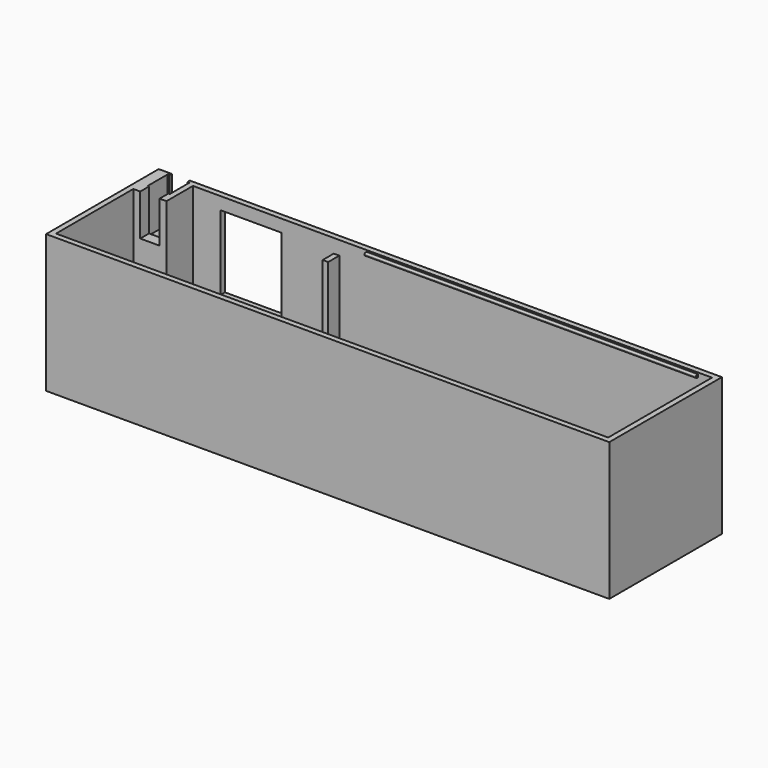
from build123d import *

# Parameters (mm, degrees)
F1_DEPTH  = 2
F0_W      = 204
F0_H      = 51
F0_W_2    = 12
F0_H_2    = 12
F2_DEPTH  = 50
F0_W_3    = 2
F0_H_3    = 37
F3_DEPTH  = 7
F0_H_4    = 5
F4_DEPTH  = 45
F6_DEPTH  = 16
F5_W      = 7
F5_H      = 4
F7_DEPTH  = 15
F8_W      = 22
F8_H      = 27
F9_DEPTH  = 5
F10_W     = 120
F10_H     = 1
F11_DEPTH = 3
F12_W     = 120
F12_H     = 1
F13_DEPTH = 3
F14_R     = 0.4


# Not quite as in the source:
# - a feature names something its author has since deleted; it is built from what else it names


with BuildPart() as f1:
    # F0 (on Top) → F1 (new body)
    with BuildSketch(Plane.XY):
        Polygon((200, 0), (65, 0), (65, -5), (65, -42), (65, -47), (200, -47), align=None)
    extrude(amount=F1_DEPTH)


with BuildPart() as f1b:
    # F0 (on Top) → F1, piece 2 (new body)
    with BuildSketch(Plane.XY):
        Polygon((63, 0), (12, 0), (12, -12), (0, -12), (0, -47), (63, -47), (63, -42), (63, -5), align=None)
    extrude(amount=F1_DEPTH)


with BuildPart() as f2:
    # F0 (on Top) → F2 (new body)
    with BuildSketch(Plane.XY):
        with Locations((100, -23.5)):
            Rectangle(F0_W, F0_H)
        Polygon((0, -12), (0, 0), (12, 0), (63, 0), (65, 0), (200, 0), (200, -47), (65, -47), (63, -47), (0, -47), align=None, mode=Mode.SUBTRACT)
        with Locations((6, -6)):
            Rectangle(F0_W_2, F0_H_2)
    extrude(amount=F2_DEPTH)

    # F5 (on face) → F6 (cut)
    with BuildSketch(Plane.XY.offset(50)):
        Polygon((9.25, 1), (2.75, 1), (2, 1), (2, -8), (2.5, -8), (9.5, -8), (10, -8), (10, 1), align=None)
    extrude(amount=-F6_DEPTH, mode=Mode.SUBTRACT)

    # F5 (on face) → F7 (cut)
    with BuildSketch(Plane.XY.offset(50)):
        with Locations((6, -10)):
            Rectangle(F5_W, F5_H)
    extrude(amount=-F7_DEPTH, mode=Mode.SUBTRACT)

    # F8 (on face) → F9 (cut)
    with BuildSketch(Plane(origin=(0, 2, 0), x_dir=(-1, 0, 0), z_dir=(0, 1, 0))):
        Polygon((-7.265019957, 34), (-4.765019957, 34), (-2.765019957, 36), (-2.765019957, 50), (-9.265019957, 50), (-9.265019957, 36), align=None)
        with Locations((-33, 32)):
            Rectangle(F8_W, F8_H)
    extrude(amount=-F9_DEPTH, mode=Mode.SUBTRACT)

    # F10 (on face) → F11 (join)
    with BuildSketch(Plane.XZ.offset(49)):
        with Locations((135, 49)):
            Rectangle(F10_W, F10_H)
    extrude(amount=-F11_DEPTH)

    # F12 (on face) → F13 (join)
    with BuildSketch(Plane(origin=(0, 2, 0), x_dir=(-1, 0, 0), z_dir=(0, 1, 0))):
        with Locations((-135, 49)):
            Rectangle(F12_W, F12_H)
    extrude(amount=-F13_DEPTH)

    # F14
    f14_edges = [f2.edges().sort_by_distance(p)[0] for p in [
        (135, -46, 48.5),
        (135, -46, 49.5),
        (135, -1, 49.5),
        (135, -1, 48.5),
    ]]
    fillet(f14_edges, radius=F14_R)


with BuildPart() as f3:
    # F0 (on Top) → F3 (new body)
    with BuildSketch(Plane.XY):
        with Locations((64, -23.5)):
            Rectangle(F0_W_3, F0_H_3)
    extrude(amount=F3_DEPTH)


with BuildPart() as f4:
    # F0 (on Top) → F4 (new body)
    with BuildSketch(Plane.XY):
        with Locations((64, -44.5)):
            Rectangle(F0_W_3, F0_H_4)
    extrude(amount=F4_DEPTH)


with BuildPart() as f4b:
    # F0 (on Top) → F4, piece 2 (new body)
    with BuildSketch(Plane.XY):
        with Locations((64, -2.5)):
            Rectangle(F0_W_3, F0_H_4)
    extrude(amount=F4_DEPTH)


solid = Compound([f1.part, f1b.part, f2.part, f3.part, f4.part, f4b.part])
